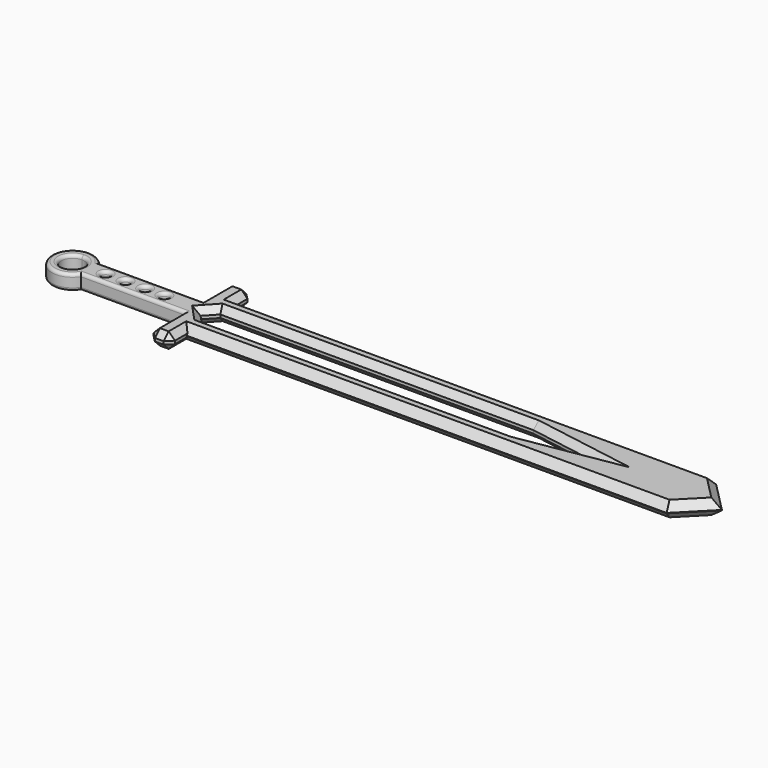
from build123d import *

# Parameters (mm, degrees)
F0_R         = 6.9707118022
F1_DEPTH     = 25
F2_R         = 5
F3_SIZE      = 10
F4_T1_DEPTH  = 805.523911048
F4_T3_DEPTH  = 132.5471516201
F4_T5_DEPTH  = 132.5471516201
F4_T10_DEPTH = 41.2459483038
F4_T15_DEPTH = 41.2459483038
F4_T20_DEPTH = 41.2459483038
F4_T25_DEPTH = 41.2459483038


# Not quite as in the source:
# - a fillet or chamfer that OpenCascade refuses, or shapes differently, is made with other operations: its cross-section is extruded or revolved along the edge and cut away or added
# - a feature names something its author has since deleted; it is built from what else it names


with BuildPart() as f1:
    # F0 (on Top) → F1 (new body)
    with BuildSketch(Plane.XY):
        with BuildLine():
            Line((-98.5221043229, 6.0890647583), (-98.5221043229, 24.5383027941))
            Line((-98.5221043229, 24.5383027941), (-259.7091133391, 24.5383027941))
            ThreePointArc((-259.7091133391, 24.5383027941), (-255.5801081547, 15.7213641607), (-254.1638105515, 6.0890647583))
            ThreePointArc((-254.1638105515, 6.0890647583), (-255.5801081547, -3.5432346441), (-259.7091133391, -12.3601732776))
            Line((-259.7091133391, -12.3601732776), (-98.5221043229, -12.3601732776))
            Line((-98.5221043229, -12.3601732776), (-98.5221043229, 6.0890647583))
        make_face()
        with Locations((-234.4832122326, 6.0890647583)):
            Circle(F0_R, mode=Mode.SUBTRACT)
        with Locations((-202.3964226246, 6.0890647583)):
            Circle(F0_R, mode=Mode.SUBTRACT)
        with Locations((-170.6961989403, 6.0890647583)):
            Circle(F0_R, mode=Mode.SUBTRACT)
        with Locations((-139.769166708, 6.0890647583)):
            Circle(F0_R, mode=Mode.SUBTRACT)
        with BuildLine():
            Line((-287.6267954707, 24.5383027941), (-259.7091133391, 24.5383027941))
            ThreePointArc((-259.7091133391, 24.5383027941), (-321.08978039, 6.0890647583), (-259.7091133391, -12.3601732776))
            Line((-259.7091133391, -12.3601732776), (-287.6267954707, -12.3601732776))
            ThreePointArc((-287.6267954707, -12.3601732776), (-306.0760335065, 6.0890647583), (-287.6267954707, 24.5383027941))
        make_face()
        with BuildLine():
            ThreePointArc((-254.1638105515, 6.0890647583), (-255.5801081547, 15.7213641607), (-259.7091133391, 24.5383027941))
            Line((-259.7091133391, 24.5383027941), (-287.6267954707, 24.5383027941))
            ThreePointArc((-287.6267954707, 24.5383027941), (-274.5812141479, 19.1346460811), (-269.1775574349, 6.0890647583))
            ThreePointArc((-269.1775574349, 6.0890647583), (-274.5812141479, -6.9565165646), (-287.6267954707, -12.3601732776))
            Line((-287.6267954707, -12.3601732776), (-259.7091133391, -12.3601732776))
            ThreePointArc((-259.7091133391, -12.3601732776), (-255.5801081547, -3.5432346441), (-254.1638105515, 6.0890647583))
        make_face()
        Polygon((-98.5221043229, 89.1931504011), (-98.5221043229, 24.5383027941), (-98.5221043229, 6.0890647583), (-81.4039707184, 6.0890647583), (-64.2858371139, 24.5383027941), (-64.2858371139, 55.9501238167), (-64.2858371139, 89.1931504011), align=None)
        Polygon((-64.2858371139, 55.9501238167), (-64.2858371139, 24.5383027941), (0, 24.5383027941), (220.2266380191, 24.5383027941), (440.4532760382, 24.5383027941), (550.5665950477, 6.0890647583), (759.2020183802, 6.0890647583), (709.9921256304, 55.9501238167), align=None)
        Polygon((0, -12.3601732776), (-64.2858371139, -12.3601732776), (-64.2858371139, -43.7719943002), (709.9921256304, -43.7719943002), (759.2020183802, 6.0890647583), (550.5665950477, 6.0890647583), (440.4532760382, -12.3601732776), (220.2266380191, -12.3601732776), align=None)
        Polygon((-81.4039707184, 6.0890647583), (-98.5221043229, 6.0890647583), (-98.5221043229, -12.3601732776), (-98.5221043229, -77.0150208846), (-64.2858371139, -77.0150208846), (-64.2858371139, -43.7719943002), (-64.2858371139, -12.3601732776), align=None)
    extrude(amount=F1_DEPTH)

    # F2
    f2_edges = [f1.edges().sort_by_distance(p)[0] for p in [
        (-179.115609, 24.538303, 25),
        (-179.115609, -12.360173, 25),
        (-287.626795, 24.538303, 25),
        (-321.08978, 6.089065, 25),
        (-321.08978, 6.089065, 0),
        (-287.626795, 24.538303, 0),
        (-179.115609, 24.538303, 0),
        (-179.115609, -12.360173, 0),
        (-241.453924, 6.089065, 0),
        (-209.367134, 6.089065, 0),
        (-177.666911, 6.089065, 0),
        (-146.739879, 6.089065, 0),
        (-177.666911, 6.089065, 25),
        (-146.739879, 6.089065, 25),
        (-209.367134, 6.089065, 25),
        (-241.453924, 6.089065, 25),
    ]]
    fillet(f2_edges, radius=F2_R)

    # F3
    f3_edges = [f1.edges().sort_by_distance(p)[0] for p in [
        (-98.522104, 56.865727, 25),
        (-98.522104, -44.687597, 25),
        (-98.522104, 56.865727, 0),
        (-98.522104, -44.687597, 0),
        (-81.403971, -77.015021, 0),
        (-81.403971, 89.19315, 25),
        (-81.403971, 89.19315, 0),
        (-98.522104, 89.19315, 12.5),
        (-81.403971, -77.015021, 25),
        (-98.522104, -77.015021, 12.5),
        (188.083719, -12.360173, 25),
        (188.083719, 24.538303, 25),
        (495.509936, -3.135554, 25),
        (495.509936, 15.313684, 25),
        (495.509936, -3.135554, 0),
        (188.083719, -12.360173, 0),
        (188.083719, 24.538303, 0),
        (495.509936, 15.313684, 0),
        (-72.844904, -3.135554, 0),
        (-72.844904, 15.313684, 0),
        (-72.844904, 15.313684, 25),
        (-72.844904, -3.135554, 25),
        (-64.285837, 72.571637, 0),
        (-64.285837, 72.571637, 25),
        (-64.285837, -60.393508, 0),
        (-64.285837, -60.393508, 25),
        (-64.285837, 89.19315, 12.5),
        (-64.285837, -77.015021, 12.5),
    ]]
    chamfer(f3_edges, length=F3_SIZE)

    # F4: chamfer of 12.15 on 8 edges, made by hand

    # F4_s2 → F4_t1 (cut)
    with BuildSketch(Plane.YZ.offset(-64.2858371139)):
        Polygon((-31.6219943002, 25), (-43.7719943002, 12.85), (-43.7719943002, 25), align=None)
        Polygon((-31.6219943002, 0), (-43.7719943002, 12.15), (-43.7719943002, 0), align=None)
        Polygon((43.8001238167, 25), (55.9501238167, 12.85), (55.9501238167, 25), align=None)
        Polygon((43.8001238167, 0), (55.9501238167, 12.15), (55.9501238167, 0), align=None)
    extrude(amount=F4_T1_DEPTH, mode=Mode.SUBTRACT)

    # F4_s4 → F4_t3 (cut)
    with BuildSketch(Plane(origin=(306.4970452709, 310.5527450182, 0), x_dir=(0, 0, 1), z_dir=(0.7024439885, 0.7117390273, 0))):
        Polygon((25, 523.9264791351), (12.85, 536.0764791351), (25, 536.0764791351), align=None)
        Polygon((0, 523.9264791351), (12.15, 536.0764791351), (0, 536.0764791351), align=None)
    extrude(amount=F4_T3_DEPTH, mode=Mode.SUBTRACT)

    # F4_s6 → F4_t5 (cut)
    with BuildSketch(Plane(origin=(393.5154564488, -398.7226209611, 0), x_dir=(0, 0, 1), z_dir=(-0.7024439885, 0.7117390273, 0))):
        Polygon((25, 532.4809330058), (12.85, 544.6309330058), (25, 544.6309330058), align=None)
        Polygon((0, 532.4809330058), (12.15, 544.6309330058), (0, 544.6309330058), align=None)
    extrude(amount=F4_T5_DEPTH, mode=Mode.SUBTRACT)


with BuildPart() as f4_tool8:
    # F4_s9 → F4_t10 (new body)
    with BuildSketch(Plane.YZ.offset(-64.2858371139)):
        Polygon((43.8001238167, 0), (55.9501238167, 12.15), (55.9501238167, 0), align=None)
    extrude(amount=-F4_T10_DEPTH)

    split(bisect_by=Plane(origin=(-37.1429185569, 0, 37.1429185569), x_dir=(0, 1, 0), z_dir=(0.7071067812, 0, -0.7071067812)), keep=Keep.TOP)


with BuildPart() as f1_1:
    add(f1.part)

    # F4_t7: cut F4_tool8
    add(f4_tool8.part, mode=Mode.SUBTRACT)


with BuildPart() as f4_tool13:
    # F4_s14 → F4_t15 (new body)
    with BuildSketch(Plane.YZ.offset(-64.2858371139)):
        Polygon((43.8001238167, 25), (55.9501238167, 12.85), (55.9501238167, 25), align=None)
    extrude(amount=-F4_T15_DEPTH)

    split(bisect_by=Plane(origin=(-24.6429185569, 0, -24.6429185569), x_dir=(0, 1, 0), z_dir=(0.7071067812, 0, 0.7071067812)), keep=Keep.TOP)


with BuildPart() as f1_2:
    add(f1_1.part)

    # F4_t12: cut F4_tool13
    add(f4_tool13.part, mode=Mode.SUBTRACT)


with BuildPart() as f4_tool18:
    # F4_s19 → F4_t20 (new body)
    with BuildSketch(Plane.YZ.offset(-64.2858371139)):
        Polygon((-31.6219943002, 0), (-43.7719943002, 12.15), (-43.7719943002, 0), align=None)
    extrude(amount=-F4_T20_DEPTH)

    split(bisect_by=Plane(origin=(-37.1429185569, 0, 37.1429185569), x_dir=(0, 1, 0), z_dir=(0.7071067812, 0, -0.7071067812)), keep=Keep.TOP)


with BuildPart() as f1_3:
    add(f1_2.part)

    # F4_t17: cut F4_tool18
    add(f4_tool18.part, mode=Mode.SUBTRACT)


with BuildPart() as f4_tool23:
    # F4_s24 → F4_t25 (new body)
    with BuildSketch(Plane.YZ.offset(-64.2858371139)):
        Polygon((-31.6219943002, 25), (-43.7719943002, 12.85), (-43.7719943002, 25), align=None)
    extrude(amount=-F4_T25_DEPTH)

    split(bisect_by=Plane(origin=(-24.6429185569, 0, -24.6429185569), x_dir=(0, 1, 0), z_dir=(0.7071067812, 0, 0.7071067812)), keep=Keep.TOP)


with BuildPart() as f1_4:
    add(f1_3.part)

    # F4_t22: cut F4_tool23
    add(f4_tool23.part, mode=Mode.SUBTRACT)


solid = f1_4.part
